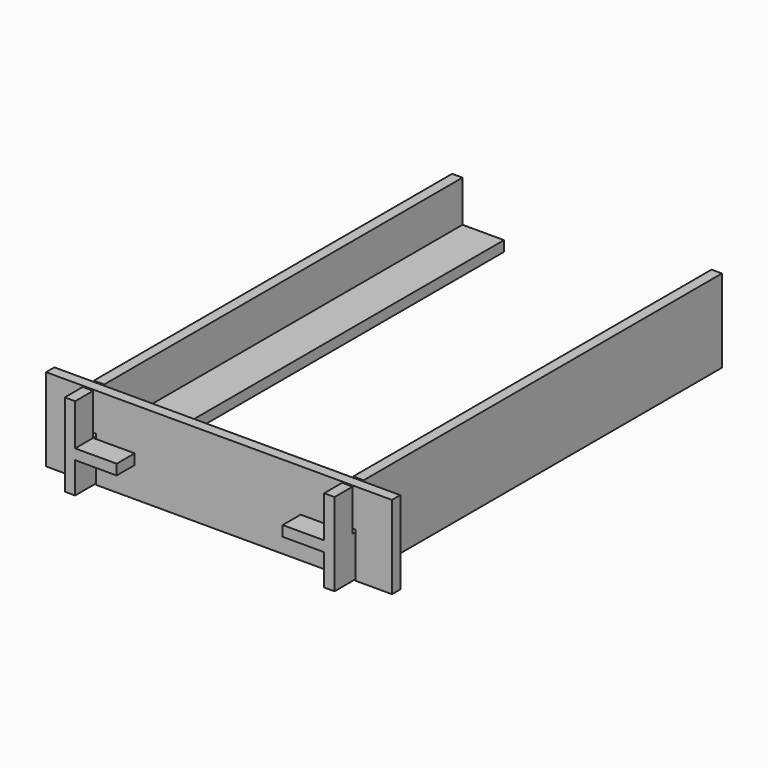
from build123d import *

# Parameters (mm, degrees)
F0_W          = 12
F0_H          = 3
F1_DEPTH      = 70
F1_DEPTH_BACK = 70
F5_DEPTH      = 3
F6_W          = 4
F6_H          = 12
F7_DEPTH      = 3
F8_W          = 4
F8_H          = 12
F9_DEPTH      = 3
F10_W         = 12
F10_H         = 4
F11_DEPTH     = 3
F12_W         = 12
F12_H         = 4
F13_DEPTH     = 3


with BuildPart() as f1:
    # F0 (on Front) → F1 (new body, two sides)
    with BuildSketch(Plane.XZ) as f1_sk:
        Polygon((36, 9), (36, 0), (39, 0), (39, 24), (36, 24), (36, 12), align=None)
        with Locations((30, 10.5)):
            Rectangle(F0_W, F0_H)
    extrude(amount=F1_DEPTH)
    extrude(f1_sk.sketch, amount=-F1_DEPTH_BACK)


with BuildPart() as f2_1:
    # F2: instance of F1
    add(f1.part.mirror(Plane.YZ))

    # F8 (on face) → F9 (cut, through all)
    with BuildSketch(Plane(origin=(-39, 0, 0), x_dir=(0, -1, 0), z_dir=(-1, 0, 0))):
        with Locations((61.5, 18)):
            Rectangle(F8_W, F8_H)
    extrude(amount=-F9_DEPTH, mode=Mode.SUBTRACT)

    # F12 (on face) → F13 (cut, through all)
    with BuildSketch(Plane.XY.offset(12)):
        with Locations((-30, -61.5)):
            Rectangle(F12_W, F12_H)
    extrude(amount=-F13_DEPTH, mode=Mode.SUBTRACT)


with BuildPart() as f5:
    # F4 (on offset) → F5 (new body)
    with BuildSketch(Plane.XZ.offset(60)):
        Polygon((-50, 24), (-50, 0), (-39.5, 0), (-39.5, 13), (-35.5, 13), (-35.5, 0), (35.5, 0), (35.5, 13), (39.5, 13), (39.5, 0), (50, 0), (50, 24), align=None)
    extrude(amount=F5_DEPTH)


with BuildPart() as f1_1:
    add(f1.part)

    # F6 (on face) → F7 (cut, through all)
    with BuildSketch(Plane.YZ.offset(39)):
        with Locations((-61.5, 18)):
            Rectangle(F6_W, F6_H)
    extrude(amount=-F7_DEPTH, mode=Mode.SUBTRACT)

    # F10 (on face) → F11 (cut, through all)
    with BuildSketch(Plane.XY.offset(12)):
        with Locations((30, -61.5)):
            Rectangle(F10_W, F10_H)
    extrude(amount=-F11_DEPTH, mode=Mode.SUBTRACT)


solid = Compound([f2_1.part, f5.part, f1_1.part])
